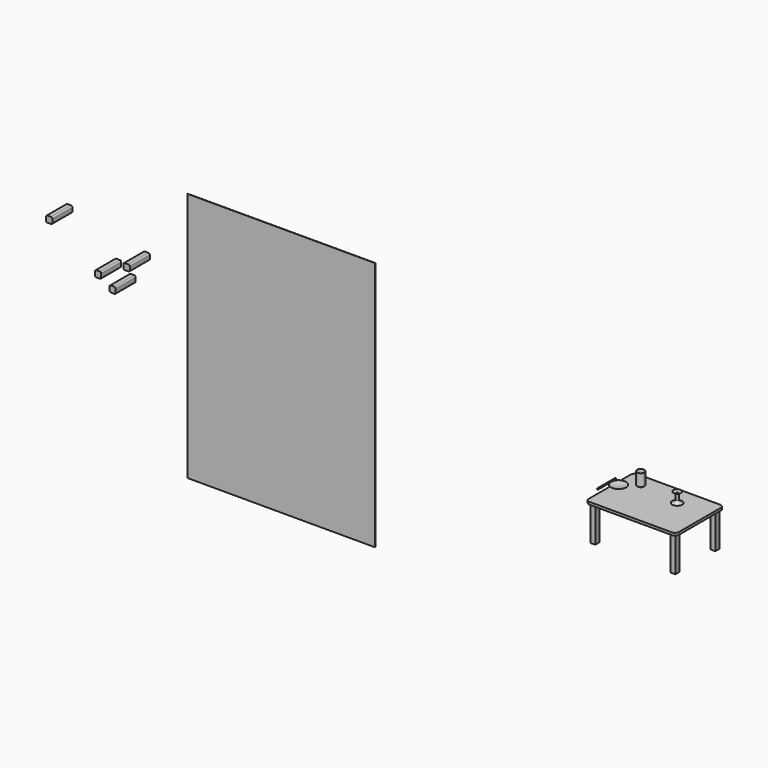
from build123d import *

# Parameters (mm, degrees)
F0_W      = 101.6
F0_H      = 101.6
F1_DEPTH  = 50.8
F2_DEPTH  = 711.2
F3_W      = 2.54
F3_H      = 215.9
F5_SIZE   = 10.16
F8_R      = 12.7
F8_R_2    = 1.27
F9_DEPTH  = 457.2
F10_DEPTH = 25.4
F11_R     = 2.54
F12_W     = 25.4
F12_H     = 115.9687861614
F14_R     = 12.7
F15_DEPTH = 101.6
F16_W     = 3810
F16_H     = 5080
F17_DEPTH = 6.35
F19_W     = 127
F19_H     = 127
F20_DEPTH = 508
F21_R     = 25.4
F22_W     = 127
F22_H     = 127
F23_DEPTH = 508
F25_W     = 127
F25_H     = 127
F26_DEPTH = 508
F27_R     = 25.4
F28_W     = 127
F28_H     = 127
F29_DEPTH = 508
F30_R     = 25.4
F30_2_R   = 25.4


# Not quite as in the source:
# - a feature of the source that left no trace in its solid (it failed there, or was rolled back) is left out


with BuildPart() as f1:
    # F0 (on Top) → F1 (new body)
    with BuildSketch(Plane.XY):
        with BuildLine():
            Line((838.2, 609.6), (-838.2, 609.6))
            ThreePointArc((-838.2, 609.6), (-892.0815367264, 587.2815367264), (-914.4, 533.4))
            Line((-914.4, 533.4), (-914.4, -533.4))
            ThreePointArc((-914.4, -533.4), (-892.0815367264, -587.2815367264), (-838.2, -609.6))
            Line((-838.2, -609.6), (838.2, -609.6))
            ThreePointArc((838.2, -609.6), (892.0815367264, -587.2815367264), (914.4, -533.4))
            Line((914.4, -533.4), (914.4, 533.4))
            ThreePointArc((914.4, 533.4), (892.0815367264, 587.2815367264), (838.2, 609.6))
        make_face()
        with Locations((-812.8, -508)):
            Rectangle(F0_W, F0_H, mode=Mode.SUBTRACT)
        with Locations((812.8, -508)):
            Rectangle(F0_W, F0_H, mode=Mode.SUBTRACT)
        with Locations((-812.8, 508)):
            Rectangle(F0_W, F0_H, mode=Mode.SUBTRACT)
        with Locations((812.8, 508)):
            Rectangle(F0_W, F0_H, mode=Mode.SUBTRACT)
        with Locations((-812.8, -508)):
            Rectangle(F0_W, F0_H)
        with Locations((812.8, -508)):
            Rectangle(F0_W, F0_H)
        with Locations((812.8, 508)):
            Rectangle(F0_W, F0_H)
        with Locations((-812.8, 508)):
            Rectangle(F0_W, F0_H)
    extrude(amount=F1_DEPTH)

    # F0 (on Top) → F2 (join)
    with BuildSketch(Plane.XY):
        with Locations((-812.8, -508)):
            Rectangle(F0_W, F0_H)
        with Locations((-812.8, 508)):
            Rectangle(F0_W, F0_H)
        with Locations((812.8, 508)):
            Rectangle(F0_W, F0_H)
        with Locations((812.8, -508)):
            Rectangle(F0_W, F0_H)
    extrude(amount=-F2_DEPTH)


with BuildPart() as f4:
    # F3 (on Front) → F4 (revolve)
    with BuildSketch(Plane.XZ):
        Polygon((-286.3245010376, 316.2632285118), (-286.3245010376, 278.1632285118), (-210.1245010376, 278.1632285118), (-210.1245010376, 316.2632285118), (-212.6645010376, 316.2632285118), align=None)
        with Locations((-211.3945010376, 424.2132285118)):
            Rectangle(F3_W, F3_H)
    revolve(axis=Axis((-286.3245010376, 0, 405.1632285118), (0, 0, 1)))

    # F5
    f5_edges = [f4.edges().sort_by_distance(p)[0] for p in [
        (-362.524501, 0, 278.163229),
    ]]
    chamfer(f5_edges, length=F5_SIZE)


with BuildPart() as f7:
    # F6 (on Front) → F7 (revolve)
    with BuildSketch(Plane.XZ):
        Polygon((-787.6298852921, 117.0304474873), (-736.8298852921, 117.0304474873), (-736.8298852921, 119.5704474873), (-889.2298852921, 144.2540854383), align=None)
    revolve(axis=Axis((-736.8298852921, 0, 187.9355122422), (0, 0, 1)))


with BuildPart() as f9:
    # F8 (on Front) → F9 (new body)
    with BuildSketch(Plane.XZ):
        with Locations((-1161.6646051407, -71.9066634774)):
            Circle(F8_R)
        with Locations((-1161.6646051407, -71.9066634774)):
            Circle(F8_R_2, mode=Mode.SUBTRACT)
        with Locations((-1161.6646051407, -71.9066634774)):
            Circle(F8_R_2)
    extrude(amount=-F9_DEPTH)

    # F8 (on Front) → F10 (join)
    with BuildSketch(Plane.XZ):
        with Locations((-1161.6646051407, -71.9066634774)):
            Circle(F8_R_2)
    extrude(amount=F10_DEPTH)

    # F11
    f11_edges = [f9.edges().sort_by_distance(p)[0] for p in [
        (-1174.364605, 0, -71.906663),
    ]]
    fillet(f11_edges, radius=F11_R)


with BuildPart() as f13:
    # F12 (on Front) → F13 (revolve)
    with BuildSketch(Plane.XZ):
        Polygon((428.1756336873, 376.7006152139), (453.5756336873, 376.7006152139), (453.5756336873, 389.4006152139), (437.0656336873, 389.4006152139), (420.5556336873, 389.4006152139), (420.5556336873, 376.7006152139), align=None)
        with Locations((440.8756336873, 318.7162221332)):
            Rectangle(F12_W, F12_H)
        with BuildLine():
            Line((351.9756336873, 205.7550829578), (453.5756336873, 205.7550829578))
            Line((453.5756336873, 205.7550829578), (453.5756336873, 260.7318290524))
            Line((453.5756336873, 260.7318290524), (428.1756336873, 260.7318290524))
            ThreePointArc((428.1756336873, 260.7318290524), (398.9567006482, 220.9339369722), (351.9756336873, 205.7550829578))
        make_face()
        with BuildLine():
            Line((420.5556336873, 389.4006152139), (437.0656336873, 389.4006152139))
            Line((437.0656336873, 389.4006152139), (375.645477209, 408.9550829578))
            ThreePointArc((375.645477209, 408.9550829578), (396.0643119403, 394.5012700165), (420.5556336873, 389.4006152139))
        make_face()
    revolve(axis=Axis((453.5756336873, 0, 307.3550829578), (0, 0, 1)))

    # F14 (on face) → F15 (cut)
    with BuildSketch(Plane.XY.offset(389.4006152139)):
        with Locations((453.5756336873, 0)):
            Circle(F14_R)
    extrude(amount=-F15_DEPTH, mode=Mode.SUBTRACT)


with BuildPart() as f17:
    # F16 (on Front) → F17 (new body)
    with BuildSketch(Plane.XZ):
        with Locations((-7580.5585479736, -39.7266790259)):
            Rectangle(F16_W, F16_H)
    extrude(amount=F17_DEPTH)


with BuildPart() as f20:
    # F19 (on face) → F20 (new body)
    with BuildSketch(Plane.XZ.offset(6.35)):
        with Locations((-11885.6859207153, 1462.1543058495)):
            Rectangle(F19_W, F19_H)
    extrude(amount=F20_DEPTH)

    # F21
    f21_edges = [f20.edges().sort_by_distance(p)[0] for p in [
        (-11822.185921, -260.35, 1525.654306),
        (-11949.185921, -260.35, 1525.654306),
        (-11949.185921, -260.35, 1398.654306),
        (-11822.185921, -260.35, 1398.654306),
    ]]
    fillet(f21_edges, radius=F21_R)


with BuildPart() as f23:
    # F22 (on offset) → F23 (new body)
    with BuildSketch(Plane.XZ.offset(31.75)):
        with Locations((-10293.2963371277, 1141.2770350553)):
            Rectangle(F22_W, F22_H)
    extrude(amount=F23_DEPTH)

    # F30#2
    f30_2_edges = [f23.edges().sort_by_distance(p)[0] for p in [
        (-10229.796337, -285.75, 1204.777035),
        (-10356.796337, -285.75, 1204.777035),
        (-10356.796337, -285.75, 1077.777035),
        (-10229.796337, -285.75, 1077.777035),
    ]]
    fillet(f30_2_edges, radius=F30_2_R)


with BuildPart() as f26:
    # F25 (on offset) → F26 (new body)
    with BuildSketch(Plane.XZ.offset(31.75)):
        with Locations((-10872.6787567139, 824.5164741749)):
            Rectangle(F25_W, F25_H)
    extrude(amount=F26_DEPTH)

    # F27
    f27_edges = [f26.edges().sort_by_distance(p)[0] for p in [
        (-10809.178757, -285.75, 761.016474),
        (-10809.178757, -285.75, 888.016474),
        (-10936.178757, -285.75, 888.016474),
        (-10936.178757, -285.75, 761.016474),
    ]]
    fillet(f27_edges, radius=F27_R)


with BuildPart() as f29:
    # F28 (on offset) → F29 (new body)
    with BuildSketch(Plane.XZ.offset(31.75)):
        with Locations((-10578.0310630798, 648.4456999137)):
            Rectangle(F28_W, F28_H)
    extrude(amount=F29_DEPTH)

    # F30
    f30_edges = [f29.edges().sort_by_distance(p)[0] for p in [
        (-10514.531063, -285.75, 711.9457),
        (-10641.531063, -285.75, 711.9457),
        (-10641.531063, -285.75, 584.9457),
        (-10514.531063, -285.75, 584.9457),
    ]]
    fillet(f30_edges, radius=F30_R)


solid = Compound([f1.part, f4.part, f7.part, f9.part, f13.part, f17.part, f20.part, f23.part, f26.part, f29.part])
